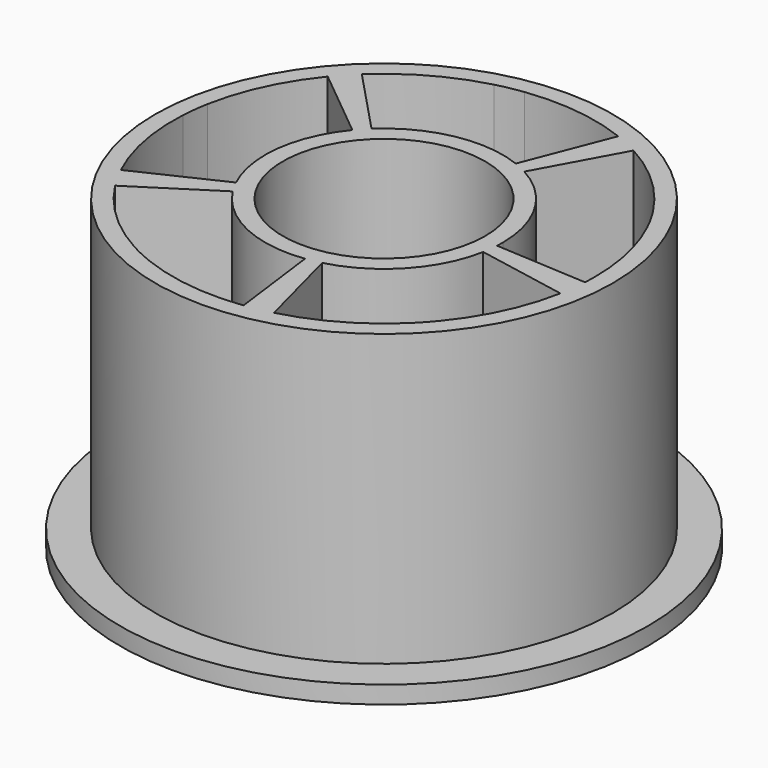
from build123d import *

# Parameters (mm, degrees)
F0_R     = 26
F0_R_2   = 11.5
F1_DEPTH = 35
F0_R_3   = 30
F2_DEPTH = 2


with BuildPart() as f1:
    # F0 (on Top) → F1 (new body)
    with BuildSketch(Plane.XY):
        with Locations((2.413794294, 2.9527412442)):
            Circle(F0_R)
        with BuildLine():
            ThreePointArc((11.1447409527, 25.3082902297), (12.5504756443, 24.7069980967), (13.9150715606, 24.0174183421))
            ThreePointArc((13.9150715606, 24.0174183421), (18.7767862132, 20.5098621771), (22.6175405184, 15.9068386076))
            ThreePointArc((22.6175405184, 15.9068386076), (23.4013731254, 14.5941129329), (24.1000296021, 13.2341418376))
            ThreePointArc((24.1000296021, 13.2341418376), (25.8282091639, 8.2220083947), (26.413794294, 2.9527412442))
            ThreePointArc((26.413794294, 2.9527412442), (26.4036425051, 2.2547564238), (26.3731957266, 1.5573620862))
            ThreePointArc((26.3731957266, 1.5573620862), (26.2357288345, 0.0346194598), (26.001582844, -1.4762802416))
            ThreePointArc((26.001582844, -1.4762802416), (24.1680511465, -7.1839401061), (20.9771739376, -12.259127024))
            ThreePointArc((20.9771739376, -12.259127024), (19.9709152269, -13.410250675), (18.8934025792, -14.4949666501))
            ThreePointArc((18.8934025792, -14.4949666501), (14.0551659828, -18.0348375872), (8.4905720708, -20.2651994882))
            ThreePointArc((8.4905720708, -20.2651994882), (6.9998781675, -20.6050140543), (5.4905720708, -20.8492216688))
            ThreePointArc((5.4905720708, -20.8492216688), (-0.5043274904, -20.8691932963), (-6.3171523646, -19.4028077413))
            ThreePointArc((-6.3171523646, -19.4028077413), (-7.7228870563, -18.8015156083), (-9.0874829725, -18.1119358537))
            ThreePointArc((-9.0874829725, -18.1119358537), (-13.9491976252, -14.6043796887), (-17.7899519304, -10.0013561192))
            ThreePointArc((-17.7899519304, -10.0013561192), (-18.5758384098, -8.6849268624), (-19.2760681095, -7.3210053419))
            ThreePointArc((-19.2760681095, -7.3210053419), (-21.1447698834, -1.6291856319), (-21.5456071385, 4.3481204022))
            ThreePointArc((-21.5456071385, 4.3481204022), (-21.4081402465, 5.8708630286), (-21.173994256, 7.38176273))
            ThreePointArc((-21.173994256, 7.38176273), (-19.3404625584, 13.0894225945), (-16.1495853495, 18.1646095124))
            ThreePointArc((-16.1495853495, 18.1646095124), (-15.1433266389, 19.3157331634), (-14.0658139912, 20.4004491385))
            ThreePointArc((-14.0658139912, 20.4004491385), (-9.2275773947, 23.9403200756), (-3.6629834828, 26.1706819766))
            ThreePointArc((-3.6629834828, 26.1706819766), (-2.1722895795, 26.5104965427), (-0.6629834828, 26.7547041572))
            ThreePointArc((-0.6629834828, 26.7547041572), (5.3319160784, 26.7746757847), (11.1447409527, 25.3082902297))
        make_face(mode=Mode.SUBTRACT)
        with BuildLine():
            ThreePointArc((15.8909575998, 2.1678404678), (15.9080839128, 2.5601247827), (15.913794294, 2.9527412442))
            ThreePointArc((15.913794294, 2.9527412442), (14.0238723352, 9.8415791635), (8.8832627565, 14.8016221118))
            ThreePointArc((8.8832627565, 14.8016221118), (8.1156775536, 15.1895107237), (7.3249517895, 15.5277375486))
            ThreePointArc((7.3249517895, 15.5277375486), (-0.1658778848, 16.2039785996), (-6.8559853664, 12.7670769348))
            ThreePointArc((-6.8559853664, 12.7670769348), (-7.4620862307, 12.1569241988), (-8.0281067555, 11.5094171451))
            ThreePointArc((-8.0281067555, 11.5094171451), (-10.9856411994, 4.597468716), (-9.7875463248, -2.824566702))
            ThreePointArc((-9.7875463248, -2.824566702), (-9.3933232872, -3.5926368521), (-8.9508129572, -4.3339385227))
            ThreePointArc((-8.9508129572, -4.3339385227), (-3.2880889655, -9.2840282353), (4.1444817935, -10.4358628944))
            ThreePointArc((4.1444817935, -10.4358628944), (4.9934664729, -10.2984961112), (5.8319817935, -10.1073504178))
            ThreePointArc((5.8319817935, -10.1073504178), (12.2896748188, -6.2514417104), (15.6819253534, 0.4614166584))
            ThreePointArc((15.6819253534, 0.4614166584), (15.813632473, 1.3112977405), (15.8909575998, 2.1678404678))
        make_face()
        with Locations((2.413794294, 2.9527412442)):
            Circle(F0_R_2, mode=Mode.SUBTRACT)
        with BuildLine():
            ThreePointArc((7.3249517895, 15.5277375486), (8.1156775536, 15.1895107237), (8.8832627565, 14.8016221118))
            Line((8.8832627565, 14.8016221118), (13.9150715606, 24.0174183421))
            ThreePointArc((13.9150715606, 24.0174183421), (12.5504756443, 24.7069980967), (11.1447409527, 25.3082902297))
            Line((11.1447409527, 25.3082902297), (7.3249517895, 15.5277375486))
        make_face()
        with BuildLine():
            Line((26.3731957266, 1.5573620862), (15.8909575998, 2.1678404678))
            ThreePointArc((15.8909575998, 2.1678404678), (15.813632473, 1.3112977405), (15.6819253534, 0.4614166584))
            Line((15.6819253534, 0.4614166584), (26.001582844, -1.4762802416))
            ThreePointArc((26.001582844, -1.4762802416), (26.2357288345, 0.0346194598), (26.3731957266, 1.5573620862))
        make_face()
        with BuildLine():
            ThreePointArc((-8.0281067555, 11.5094171451), (-7.4620862307, 12.1569241988), (-6.8559853664, 12.7670769348))
            Line((-6.8559853664, 12.7670769348), (-14.0658139912, 20.4004491385))
            ThreePointArc((-14.0658139912, 20.4004491385), (-15.1433266389, 19.3157331634), (-16.1495853495, 18.1646095124))
            Line((-16.1495853495, 18.1646095124), (-8.0281067555, 11.5094171451))
        make_face()
        with BuildLine():
            Line((8.4905720708, -20.2651994882), (5.8319817935, -10.1073504178))
            ThreePointArc((5.8319817935, -10.1073504178), (4.9934664729, -10.2984961112), (4.1444817935, -10.4358628944))
            Line((4.1444817935, -10.4358628944), (5.4905720708, -20.8492216688))
            ThreePointArc((5.4905720708, -20.8492216688), (6.9998781675, -20.6050140543), (8.4905720708, -20.2651994882))
        make_face()
        with BuildLine():
            ThreePointArc((-8.9508129572, -4.3339385227), (-9.3933232872, -3.5926368521), (-9.7875463248, -2.824566702))
            Line((-9.7875463248, -2.824566702), (-19.2760681095, -7.3210053419))
            ThreePointArc((-19.2760681095, -7.3210053419), (-18.5758384098, -8.6849268624), (-17.7899519304, -10.0013561192))
            Line((-17.7899519304, -10.0013561192), (-8.9508129572, -4.3339385227))
        make_face()
    extrude(amount=F1_DEPTH)

    # F0 (on Top) → F2 (join)
    with BuildSketch(Plane.XY):
        with Locations((2.413794294, 2.9527412442)):
            Circle(F0_R_3)
        with Locations((2.413794294, 2.9527412442)):
            Circle(F0_R, mode=Mode.SUBTRACT)
    extrude(amount=F2_DEPTH)


solid = f1.part
